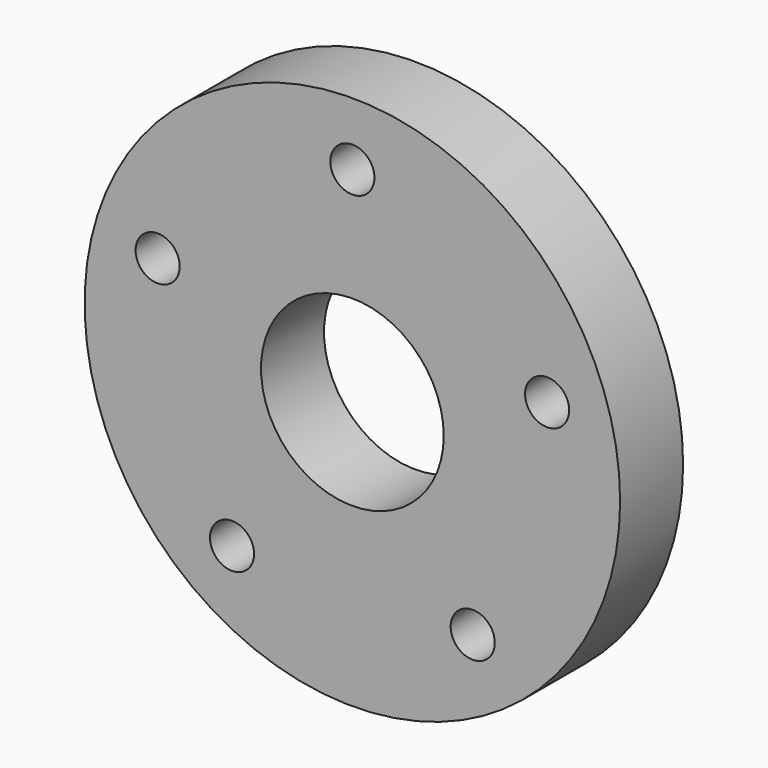
from build123d import *

# Parameters (mm, degrees)
F0_R     = 85
F0_R_2   = 7
F0_R_3   = 29
F1_DEPTH = 25


# Not quite as in the source:
# - the program builds the solid bodies; features that only make, move or delete a surface that nothing else refers to are left out


with BuildPart() as f1:
    # F0 (on Front) → F1 (new body)
    with BuildSketch(Plane.XZ):
        Circle(F0_R)
        with Locations((-38.206041399, -52.5861046344)):
            Circle(F0_R_2, mode=Mode.SUBTRACT)
        with Locations((38.206041399, -52.5861046344)):
            Circle(F0_R_2, mode=Mode.SUBTRACT)
        with Locations((-61.8186735592, 20.0861046344)):
            Circle(F0_R_2, mode=Mode.SUBTRACT)
        Circle(F0_R_3, mode=Mode.SUBTRACT)
        with Locations((61.8186735592, 20.0861046344)):
            Circle(F0_R_2, mode=Mode.SUBTRACT)
        with Locations((0, 65)):
            Circle(F0_R_2, mode=Mode.SUBTRACT)
    extrude(amount=F1_DEPTH)


solid = f1.part
